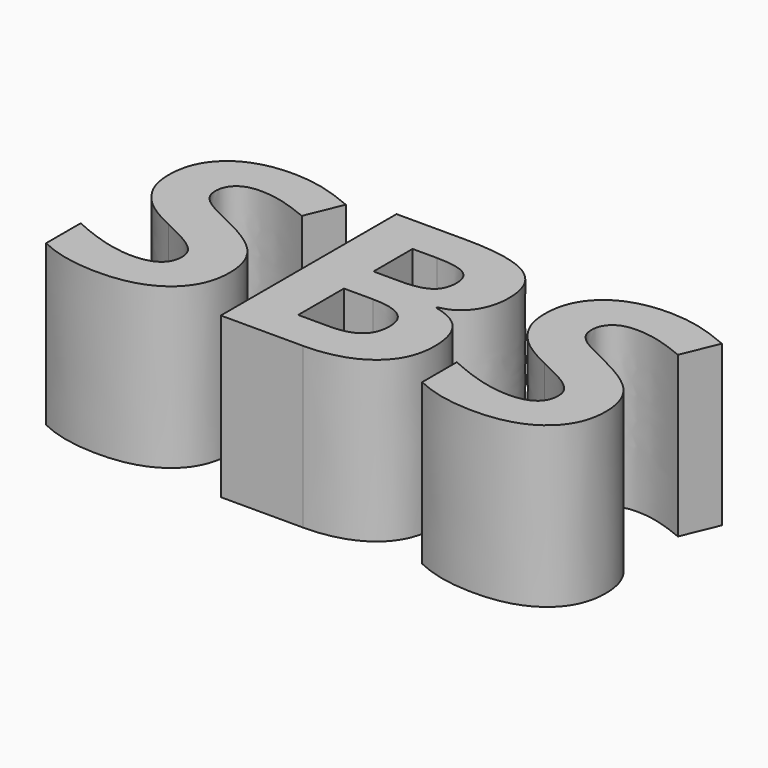
from build123d import *

# Parameters (mm, degrees)
F2_TEXT_SIZE = 19.2316016182
F3_DEPTH     = 10


# Not quite as in the source:
# - the program builds the solid bodies; features that only make, move or delete a surface that nothing else refers to are left out
# - Text() gives the source's letters only with a copy of the font that has no kerning and outlines rounded to 1/6400 em; it was checked with that copy


with BuildPart() as f3:
    # F2 (on face) → F3 (new body)
    with BuildSketch(Plane.XY.offset(15.3)):
        with Locations((-17.2639042139, -6.9183656015)):
            Text('SBS', F2_TEXT_SIZE, font='Open Sans', font_style=FontStyle.BOLD, text_align=(TextAlign.LEFT, TextAlign.BOTTOM))
    extrude(amount=F3_DEPTH)


solid = f3.part
